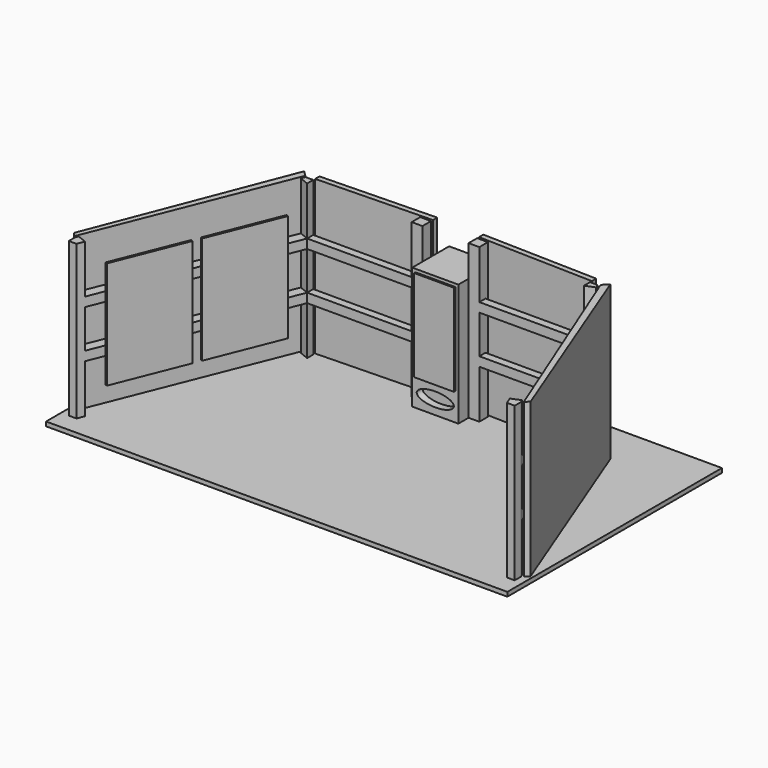
from build123d import *

# Parameters (mm, degrees)
F0_W      = 300
F0_H      = 174.4493450305
F1_DEPTH  = 2.794
F2_W      = 5
F2_H      = 5
F2_W_2    = 7
F2_H_2    = 7
F3_DEPTH  = 100
F4_W      = 30
F4_H      = 30
F5_DEPTH  = 79.6
F6_W      = 26
F6_H      = 59.6
F7_DEPTH  = 1.1
F9_DEPTH  = 4.8
F11_DEPTH = 100
F12_W     = 68
F12_H     = 5
F13_DEPTH = 100
F14_W     = 68
F14_H     = 5
F15_DEPTH = 100
F17_DEPTH = 100
F18_W     = 129.6291201784
F18_H     = 31.5
F18_H_2   = 25
F19_DEPTH = 16.5
F20_W     = 68
F20_H     = 31.5
F20_H_2   = 25
F21_DEPTH = 25
F22_W     = 68
F22_H     = 31.5
F22_H_2   = 25
F23_DEPTH = 25
F24_W     = 129.6291201784
F24_H     = 31.5
F24_H_2   = 25
F25_DEPTH = 25
F26_DEPTH = 100
F27_W     = 50
F27_H     = 16.5
F27_H_2   = 25
F27_H_3   = 6
F28_DEPTH = 1.3


with BuildPart() as f1:
    # F0 (on Top) → F1 (new body)
    with BuildSketch(Plane.XY):
        Rectangle(F0_W, F0_H)
    extrude(amount=F1_DEPTH)

    # F2 (on face) → F3 (join)
    with BuildSketch(Plane.XY.offset(2.794)):
        with Locations((-142.5, -72.5)):
            Rectangle(F2_W, F2_H)
        with Locations((-92.5, 52.5)):
            Rectangle(F2_W, F2_H)
        with Locations((92.5, 52.5)):
            Rectangle(F2_W, F2_H)
        with Locations((142.5, -72.5)):
            Rectangle(F2_W, F2_H)
        with Locations((-18.5, 53.5)):
            Rectangle(F2_W_2, F2_H_2)
        with Locations((18.5, 53.5)):
            Rectangle(F2_W_2, F2_H_2)
        Polygon((-90, 60), (-90, 56.5), (-15, 58.5), (-15, 62), align=None)
        Polygon((90, 60), (15, 62), (15, 58.5), (90, 56.5), align=None)
        Polygon((96.0606601718, 56.0606601718), (146.02977278, -68.9093268035), (148.4921801752, -66.4220492114), (99.5606601718, 59.5606601718), align=None)
        Polygon((-96.0627255066, 56.0585908075), (-99.5627255066, 59.5562038535), (-148.5355339059, -66.4644660941), (-146.0606601718, -68.9393398282), align=None)
    extrude(amount=F3_DEPTH)

    # F4 (on face) → F5 (join)
    with BuildSketch(Plane.XY.offset(2.794)):
        with Locations((0, 56.6965335608)):
            Rectangle(F4_W, F4_H)
    extrude(amount=F5_DEPTH)

    # F6 (on face) → F7 (join)
    with BuildSketch(Plane.XZ.offset(-41.6965335608)):
        with Locations((0, 50.594)):
            Rectangle(F6_W, F6_H)
    extrude(amount=F7_DEPTH)

    # F8 (on face) → F9 (cut)
    with BuildSketch(Plane.XZ.offset(-41.6965335608)):
        with BuildLine():
            add(Edge.make_bspline(
                [(12.06954394, 11.794), (12.06954394, 19.7033991149), (-6.03477197, 15.7486995575), (-24.13908788, 11.794), (-6.03477197, 7.8393004425), (12.06954394, 3.8846008851), (12.06954394, 11.794)],
                knots=[0, 0, 0, 2.0943951024, 2.0943951024, 4.1887902048, 4.1887902048, 6.2831853072, 6.2831853072, 6.2831853072], degree=2, weights=[1, 0.5, 1, 0.5, 1, 0.5, 1]))
        make_face()
    extrude(amount=-F9_DEPTH, mode=Mode.SUBTRACT)

    # F10 (on face) → F11 (join)
    with BuildSketch(Plane.XY.offset(2.794)):
        Polygon((-140, -70), (-140, -75), (-90, 50), (-95, 50), (-95, 55), (-145, -70), align=None)
    extrude(amount=F11_DEPTH)

    # F12 (on face) → F13 (join)
    with BuildSketch(Plane.XY.offset(2.794)):
        with Locations((-56, 52.5)):
            Rectangle(F12_W, F12_H)
    extrude(amount=F13_DEPTH)

    # F14 (on face) → F15 (join)
    with BuildSketch(Plane.XY.offset(2.794)):
        with Locations((56, 52.5)):
            Rectangle(F14_W, F14_H)
    extrude(amount=F15_DEPTH)

    # F16 (on face) → F17 (join)
    with BuildSketch(Plane.XY.offset(2.794)):
        Polygon((90, 50), (140, -75), (140, -70), (145, -70), (95, 55), (95, 50), align=None)
    extrude(amount=F17_DEPTH)

    # F18 (on face) → F19 (cut)
    with BuildSketch(Plane(origin=(-94.8275862069, 37.9310344828, 0), x_dir=(0.3713906764, 0.9284766909, 0), z_dir=(0.9284766909, -0.3713906764, 0))):
        with Locations((-51.8158864168, 87.044)):
            Rectangle(F18_W, F18_H)
        with Locations((-51.8158864168, 52.794)):
            Rectangle(F18_W, F18_H_2)
        with Locations((-51.8158864168, 18.544)):
            Rectangle(F18_W, F18_H)
    extrude(amount=-F19_DEPTH, mode=Mode.SUBTRACT)

    # F20 (on face) → F21 (cut)
    with BuildSketch(Plane.XZ.offset(-50)):
        with Locations((-56, 87.044)):
            Rectangle(F20_W, F20_H)
        with Locations((-56, 52.794)):
            Rectangle(F20_W, F20_H_2)
        with Locations((-56, 18.544)):
            Rectangle(F20_W, F20_H)
    extrude(amount=-F21_DEPTH, mode=Mode.SUBTRACT)

    # F22 (on face) → F23 (cut)
    with BuildSketch(Plane.XZ.offset(-50)):
        with Locations((56, 18.544)):
            Rectangle(F22_W, F22_H)
        with Locations((56, 52.794)):
            Rectangle(F22_W, F22_H_2)
        with Locations((56, 87.044)):
            Rectangle(F22_W, F22_H)
    extrude(amount=-F23_DEPTH, mode=Mode.SUBTRACT)

    # F24 (on face) → F25 (cut)
    with BuildSketch(Plane(origin=(94.8275862069, 37.9310344828, 0), x_dir=(0.3713906764, -0.9284766909, 0), z_dir=(-0.9284766909, -0.3713906764, 0))):
        with Locations((51.8158864168, 87.044)):
            Rectangle(F24_W, F24_H)
        with Locations((51.8158864168, 52.794)):
            Rectangle(F24_W, F24_H_2)
        with Locations((51.8158864168, 18.544)):
            Rectangle(F24_W, F24_H)
    extrude(amount=-F25_DEPTH, mode=Mode.SUBTRACT)

    # F2 (on face) → F26 (join)
    with BuildSketch(Plane.XY.offset(2.794)):
        Polygon((-96.0627255066, 56.0585908075), (-99.5627255066, 59.5562038535), (-148.5355339059, -66.4644660941), (-146.0606601718, -68.9393398282), align=None)
        Polygon((-90, 60), (-90, 56.5), (-15, 58.5), (-15, 62), align=None)
        Polygon((90, 60), (15, 62), (15, 58.5), (90, 56.5), align=None)
        Polygon((96.0606601718, 56.0606601718), (146.02977278, -68.9093268035), (148.4921801752, -66.4220492114), (99.5606601718, 59.5606601718), align=None)
    extrude(amount=F26_DEPTH)

    # F27 (on face) → F28 (join)
    with BuildSketch(Plane(origin=(-94.8275862069, 37.9310344828, 0), x_dir=(0.3713906764, 0.9284766909, 0), z_dir=(0.9284766909, -0.3713906764, 0))):
        with Locations((-79.630446506, 79.544)):
            Rectangle(F27_W, F27_H)
        with Locations((-79.630446506, 52.794)):
            Rectangle(F27_W, F27_H_2)
        with Locations((-79.630446506, 68.294)):
            Rectangle(F27_W, F27_H_3)
        with Locations((-79.630446506, 26.044)):
            Rectangle(F27_W, F27_H)
        with Locations((-79.630446506, 37.294)):
            Rectangle(F27_W, F27_H_3)
        with Locations((-24.0013263276, 26.044)):
            Rectangle(F27_W, F27_H)
        with Locations((-24.0013263276, 37.294)):
            Rectangle(F27_W, F27_H_3)
        with Locations((-24.0013263276, 52.794)):
            Rectangle(F27_W, F27_H_2)
        with Locations((-24.0013263276, 68.294)):
            Rectangle(F27_W, F27_H_3)
        with Locations((-24.0013263276, 79.544)):
            Rectangle(F27_W, F27_H)
    extrude(amount=F28_DEPTH)


solid = f1.part
